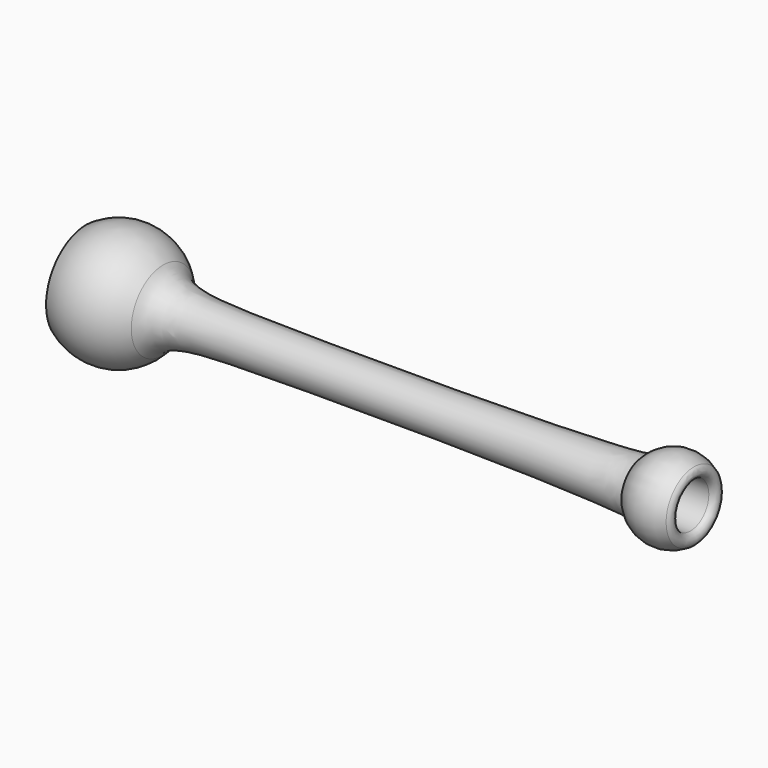
from build123d import *

# Parameters (mm, degrees)
F2_R = 2


# Not quite as in the source:
# - a fillet or chamfer that OpenCascade refuses, or shapes differently, is made with other operations: its cross-section is extruded or revolved along the edge and cut away or added


with BuildPart() as f1:
    # F0 (on Front) → F1 (revolve)
    with BuildSketch(Plane.XZ):
        with BuildLine():
            ThreePointArc((-7.0685046336, 10.3095219212), (4.6853520259, 11.5886788028), (12.2474487139, 2.5))
            Line((12.2474487139, 2.5), (74.2474487139, 2.5))
            Line((74.2474487139, 2.5), (181.4870995989, 7.242008176))
            ThreePointArc((181.4870995989, 7.242008176), (172.2166286642, 12.6424148054), (162.3323179763, 8.4703139749))
            add(Edge.make_bspline(
                [(13.7809895682, 12.3177978136), (16.8322612088, 7.285858607), (42.8552617273, 5.9648264947), (153.4052985384, 6.3755253316), (162.3323179763, 8.4703139749)],
                knots=[0, 0, 0, 0, 0.3380399349, 1, 1, 1, 1], degree=3))
            ThreePointArc((13.7809895682, 12.3177978136), (2.4835532955, 18.3159979112), (-10.003236638, 15.5428141988))
            Line((-10.003236638, 15.5428141988), (-7.0685046336, 10.3095219212))
        make_face()
    revolve(axis=Axis((35, 0, 0), (1, 0, 0)))

    # F2
    f2_edges = [f1.edges().sort_by_distance(p)[0] for p in [
        (181.4871, 0, -7.242008),
        (-7.068505, 0, -10.309522),
        (12.247449, 0, -2.5),
    ]]
    fillet(f2_edges, radius=F2_R)

    # F3: fillet of radius 5 on 1 edges, made by hand

    # F3_s1 → F3_t2 (revolve, cut)
    with BuildSketch(Plane.XZ):
        with BuildLine():
            ThreePointArc((74.3578338514, 2.5048810978), (74.2474217443, 2.5012204234), (74.136955711, 2.5))
            Line((74.136955711, 2.5), (74.136955711, 2.4))
            Line((74.136955711, 2.4), (74.249658574, 2.4))
            Line((74.249658574, 2.4), (74.3622514143, 2.4049787198))
            Line((74.3622514143, 2.4049787198), (74.3578338514, 2.5048810978))
        make_face()
    revolve(axis=Axis((74.2474487139, 0, 0), (1, 0, 0)), mode=Mode.SUBTRACT)


solid = f1.part
